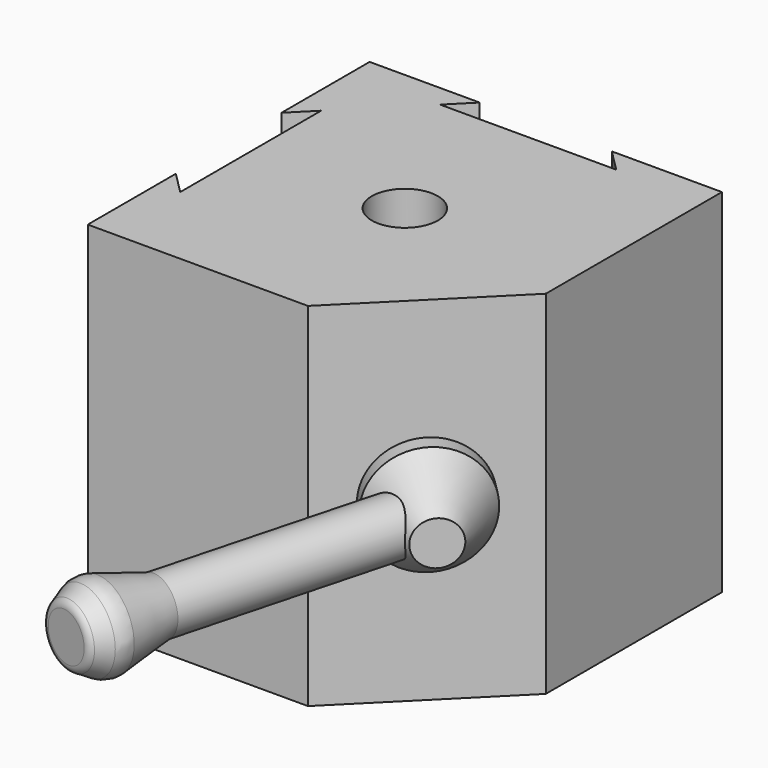
from build123d import *

# Parameters (mm, degrees)
F1_R      = 4.7625
F2_DEPTH  = 25.4
F3_DEPTH  = 19.05
F4_DEPTH  = 19.05
F5_R      = 7.9375
F6_DEPTH  = 47.1463446356
F7_DEPTH  = 34.925
F8_R      = 4.7625
F9_DEPTH  = 12.2213446356
F11_DEPTH = 50.8010001


with BuildPart() as f2:
    # F1 (on Top) → F2 (new body, symmetric)
    with BuildSketch(Plane.XY):
        Polygon((-11.8019743879, 22.225), (-12.7, 22.225), (-22.225, 12.7), (-22.225, 11.8019743879), align=None)
        Polygon((25.4, -6.35), (25.4, 25.4), (9.525, 25.4), (12.7, 22.225), (-11.8019743879, 22.225), (-22.225, 11.8019743879), (-22.225, -12.7), (-25.4, -9.525), (-25.4, -25.4), (6.35, -25.4), align=None)
        Circle(F1_R, mode=Mode.SUBTRACT)
        Polygon((-12.7, 22.225), (-9.525, 25.4), (-25.4, 25.4), (-25.4, 9.525), (-22.225, 12.7), align=None)
    extrude(amount=F2_DEPTH, both=True)

    # F1 (on Top) → F3 (cut, symmetric)
    with BuildSketch(Plane.XY):
        Polygon((-12.7, 22.225), (-9.525, 25.4), (-25.4, 25.4), (-25.4, 9.525), (-22.225, 12.7), align=None)
        Polygon((-11.8019743879, 22.225), (-12.7, 22.225), (-22.225, 12.7), (-22.225, 11.8019743879), align=None)
    extrude(amount=F3_DEPTH, both=True, mode=Mode.SUBTRACT)

    # F5 (on face) → F6 (cut, through all)
    with BuildSketch(Plane(origin=(-17.4625, 17.4625, 0), x_dir=(0.7071067812, 0.7071067812, 0), z_dir=(0.7071067812, -0.7071067812, 0))):
        Circle(F5_R)
    extrude(amount=F6_DEPTH, mode=Mode.SUBTRACT)


with BuildPart() as f4:
    # F1 (on Top) → F4 (new body, symmetric)
    with BuildSketch(Plane.XY):
        Polygon((-12.7, 22.225), (-9.525, 25.4), (-25.4, 25.4), (-25.4, 9.525), (-22.225, 12.7), align=None)
    extrude(amount=F4_DEPTH, both=True)

    # F5 (on face) → F7 (join)
    with BuildSketch(Plane(origin=(-17.4625, 17.4625, 0), x_dir=(0.7071067812, 0.7071067812, 0), z_dir=(0.7071067812, -0.7071067812, 0))):
        Circle(F5_R)
    extrude(amount=F7_DEPTH)

    # F8 (on face) → F9 (join, through all)
    with BuildSketch(Plane(origin=(7.2332043329, -7.2332043329, 0), x_dir=(0.7071067812, 0.7071067812, 0), z_dir=(0.7071067812, -0.7071067812, 0))):
        Circle(F8_R)
    extrude(amount=F9_DEPTH)

    # F10 (on face) → F11 (cut, through all)
    with BuildSketch(Plane.XY.offset(25.4)):
        with BuildLine():
            Line((4.4901280605, 2.2450640303), (2.2450640303, 4.4901280605))
            ThreePointArc((2.2450640303, 4.4901280605), (-4.4901280605, 4.4901280605), (-4.4901280605, -2.2450640303))
            Line((-4.4901280605, -2.2450640303), (-2.2450640303, -4.4901280605))
            ThreePointArc((-2.2450640303, -4.4901280605), (4.4901280605, -4.4901280605), (4.4901280605, 2.2450640303))
        make_face()
    extrude(amount=-F11_DEPTH, mode=Mode.SUBTRACT)


with BuildPart() as f13:
    # F12 (on Top) → F13 (revolve)
    with BuildSketch(Plane.XY):
        Polygon((23.3916454727, -23.3916454727), (9.1398079092, -9.1398079092), (3.5271478335, -14.7524679849), (5.2109458562, -16.4362660076), (6.2226737785, -15.4245380853), (7.9064718012, -17.108336108), (9.5902698239, -18.7921341307), (8.5785419016, -19.803862053), (11.946137947, -23.1714580984), (21.1465814424, -25.636709503), align=None)
        Polygon((6.2226737785, -15.4245380853), (5.2109458562, -16.4362660076), (7.9064718012, -17.108336108), align=None)
        Polygon((9.5902698239, -18.7921341307), (7.9064718012, -17.108336108), (8.5785419016, -19.803862053), align=None)
    revolve(axis=Axis((0, 0, 0), (0.7071067812, -0.7071067812, 0)))


with BuildPart() as f15:
    # F14 (on Top) → F15 (revolve)
    with BuildSketch(Plane.XY):
        with BuildLine():
            Line((21.9140755042, -16.6387536732), (18.8472610057, -15.817003205))
            Line((18.8472610057, -15.817003205), (5.0418531399, -67.3394867792))
            Line((5.0418531399, -67.3394867792), (8.3407770996, -68.2234307901))
            ThreePointArc((8.3407770996, -68.2234307901), (8.9981774742, -68.2234307901), (9.567502899, -67.8947306028))
            Line((9.567502899, -67.8947306028), (11.2324371661, -66.2297963357))
            ThreePointArc((11.2324371661, -66.2297963357), (11.9206906515, -65.1997522032), (12.1623731358, -63.9847323055))
            Line((12.1623731358, -63.9847323055), (12.1623731358, -56.0994168706))
            Line((12.1623731358, -56.0994168706), (21.0372781924, -22.9778202871))
            Line((21.0372781924, -22.9778202871), (20.2705745678, -22.7723826701))
            Line((20.2705745678, -22.7723826701), (21.9140755042, -16.6387536732))
        make_face()
    revolve(axis=Axis((12.8237458576, -38.2970677779, 0), (0.2588190451, 0.9659258263, 0)))


solid = Compound([f2.part, f4.part, f13.part, f15.part])
